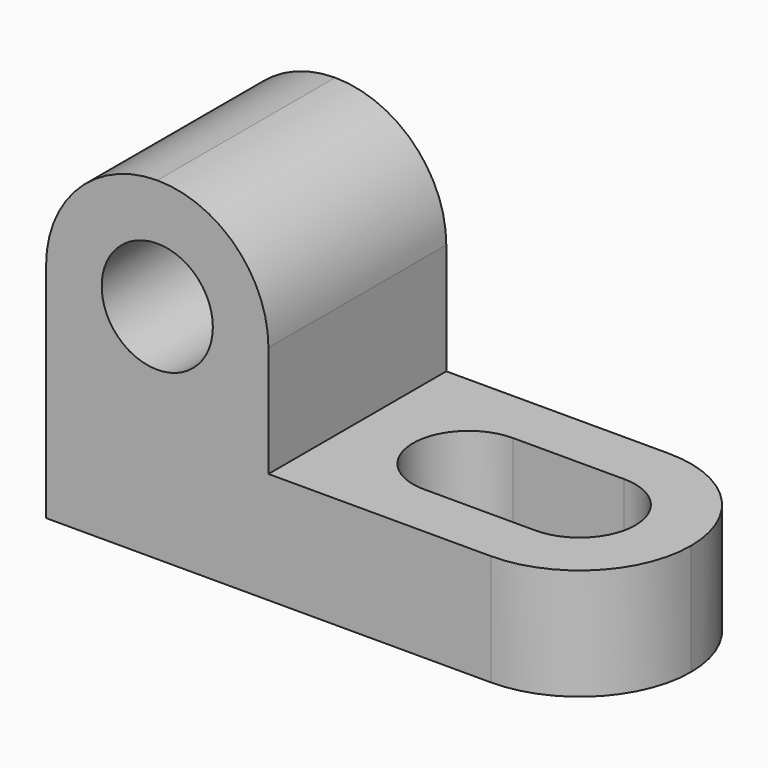
from build123d import *

# Parameters (mm, degrees)
F1_DEPTH = 25.4
F2_R     = 12.7
F3_R     = 12.69999
F4_R     = 12.7
F5_R     = 12.69999
F7_DEPTH = 25.4
F8_R     = 6.35
F9_DEPTH = 31.75


# Not quite as in the source:
# - a fillet or chamfer is up to 0.001 mm smaller than in the source, because OpenCascade refuses the exact size


with BuildPart() as f1:
    # F0 (on Front) → F1 (new body)
    with BuildSketch(Plane.XZ):
        Polygon((0, 38.1), (0, 0), (63.5, 0), (63.5, 12.7), (25.4, 12.7), (25.4, 38.1), align=None)
    extrude(amount=F1_DEPTH)

    # F2
    f2_edges = [f1.edges().sort_by_distance(p)[0] for p in [
        (63.5, -25.4, 6.35),
    ]]
    fillet(f2_edges, radius=F2_R)

    # F3 (radius 12.7 in the source; OpenCascade refuses exactly that, so slightly less here)
    f3_edges = [f1.edges().sort_by_distance(p)[0] for p in [
        (63.5, 0, 6.35),
    ]]
    fillet(f3_edges, radius=F3_R)

    # F4
    f4_edges = [f1.edges().sort_by_distance(p)[0] for p in [
        (25.4, -12.7, 38.1),
    ]]
    fillet(f4_edges, radius=F4_R)

    # F5 (radius 12.7 in the source; OpenCascade refuses exactly that, so slightly less here)
    f5_edges = [f1.edges().sort_by_distance(p)[0] for p in [
        (0, -12.7, 38.1),
    ]]
    fillet(f5_edges, radius=F5_R)

    # F6 (on face) → F7 (cut)
    with BuildSketch(Plane.XY.offset(12.7)):
        with BuildLine():
            ThreePointArc((38.3966746256, -19.0430658334), (42.6938210606, -17.0839831277), (44.45, -12.7))
            ThreePointArc((44.45, -12.7), (42.5901280605, -8.2098719395), (38.1, -6.35))
            ThreePointArc((38.1, -6.35), (31.7518177342, -12.5480726474), (37.7962322754, -19.0427301038))
            Line((37.7962322754, -19.0427301038), (38.3966746256, -19.0430658334))
        make_face()
        with BuildLine():
            ThreePointArc((50.79644948, -19.0499990074), (46.3086168165, -17.1888725866), (44.45, -12.7))
            ThreePointArc((44.45, -12.7), (42.6938210606, -17.0839831277), (38.3966746256, -19.0430658334))
            Line((38.3966746256, -19.0430658334), (50.79644948, -19.0499990074))
        make_face()
        with BuildLine():
            ThreePointArc((38.1, -6.35), (42.5901280605, -8.2098719395), (44.45, -12.7))
            ThreePointArc((44.45, -12.7), (46.3098719395, -8.2098719395), (50.8, -6.35))
            Line((50.8, -6.35), (38.1, -6.35))
        make_face()
        with BuildLine():
            ThreePointArc((50.8, -6.35), (46.3098719395, -8.2098719395), (44.45, -12.7))
            ThreePointArc((44.45, -12.7), (46.3086168165, -17.1888725866), (50.79644948, -19.0499990074))
            ThreePointArc((50.79644948, -19.0499990074), (55.2888725866, -17.1913831835), (57.15, -12.7))
            ThreePointArc((57.15, -12.7), (55.2901280605, -8.2098719395), (50.8, -6.35))
        make_face()
        with BuildLine():
            ThreePointArc((37.7962322754, -19.0427301038), (38.09644948, -19.0499990074), (38.3966746256, -19.0430658334))
            Line((38.3966746256, -19.0430658334), (37.7962322754, -19.0427301038))
        make_face()
    extrude(amount=-F7_DEPTH, mode=Mode.SUBTRACT)

    # F8 (on face) → F9 (cut)
    with BuildSketch(Plane.XZ.offset(25.4)):
        with Locations((12.7, 25.4)):
            Circle(F8_R)
    extrude(amount=-F9_DEPTH, mode=Mode.SUBTRACT)


solid = f1.part
